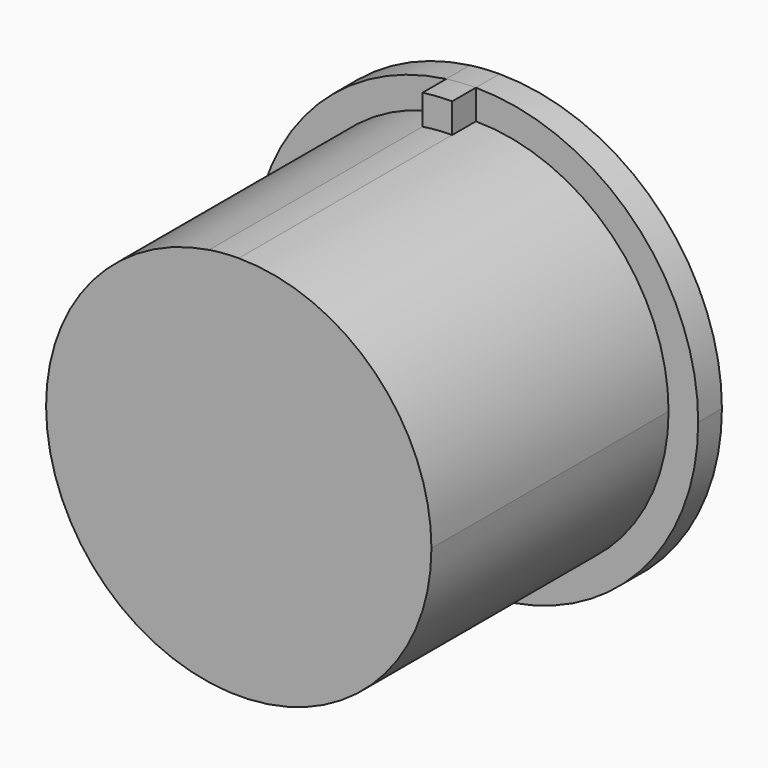
from build123d import *
from build123d import SkipClean  # not in build123d's __all__

# Parameters (mm, degrees)
F3_DEPTH = 3.175
F4_DEPTH = 31.75
F5_DEPTH = 3.175
F6_DEPTH = 3.175


# Not quite as in the source:
# - a length typed as a fraction of an inch, garbled in the dataset ("3 / 203.2 mm" for 3/8 in), is restored


with BuildPart() as f3:
    # F2 (on Front) → F3 (new body)
    with BuildSketch(Plane.XZ):
        with BuildLine():
            Line((-3.175, 23.5998841364), (-3.175, 20.3918067186))
            ThreePointArc((-3.175, 20.3918067186), (-1.5922460699, 20.5759849996), (0, 20.6375))
            Line((0, 20.6375), (0, 23.8125))
            ThreePointArc((0, 23.8125), (-1.591055507, 23.7592865765), (-3.175, 23.5998841364))
        make_face()
        with BuildLine():
            ThreePointArc((20.6375, 0), (-13.4235305294, -15.6753065161), (-3.175, 20.3918067186))
            Line((-3.175, 20.3918067186), (-3.175, 23.5998841364))
            ThreePointArc((-3.175, 23.5998841364), (-15.6753065161, -17.9253987926), (23.8125, 0))
            ThreePointArc((23.8125, 0), (16.837980227, 16.837980227), (0, 23.8125))
            Line((0, 23.8125), (0, 20.6375))
            ThreePointArc((0, 20.6375), (14.5929161967, 14.5929161967), (20.6375, 0))
        make_face()
    extrude(amount=-F3_DEPTH)

    # F2 (on Front) → F4 (join)
    with BuildSketch(Plane.XZ):
        with BuildLine():
            ThreePointArc((0, 20.6375), (-1.5922460699, 20.5759849996), (-3.175, 20.3918067186))
            ThreePointArc((-3.175, 20.3918067186), (-13.4235305294, -15.6753065161), (20.6375, 0))
            ThreePointArc((20.6375, 0), (14.5929161967, 14.5929161967), (0, 20.6375))
        make_face()
    extrude(amount=F4_DEPTH)

    # F2 (on Front) → F5 (join)
    with BuildSketch(Plane.XZ):
        with BuildLine():
            Line((-3.175, 23.5998841364), (-3.175, 20.3918067186))
            ThreePointArc((-3.175, 20.3918067186), (-1.5922460699, 20.5759849996), (0, 20.6375))
            Line((0, 20.6375), (0, 23.8125))
            ThreePointArc((0, 23.8125), (-1.591055507, 23.7592865765), (-3.175, 23.5998841364))
        make_face()
    with SkipClean():  # cleaning this boolean's faces spoils the solid; the shape is the same uncleaned
        extrude(amount=F5_DEPTH)

    # F2 (on Front) → F6 (join)
    with BuildSketch(Plane.XZ):
        with BuildLine():
            ThreePointArc((0, 20.6375), (-1.5922460699, 20.5759849996), (-3.175, 20.3918067186))
            ThreePointArc((-3.175, 20.3918067186), (-13.4235305294, -15.6753065161), (20.6375, 0))
            ThreePointArc((20.6375, 0), (14.5929161967, 14.5929161967), (0, 20.6375))
        make_face()
        with BuildLine():
            Line((-3.175, 23.5998841364), (-3.175, 20.3918067186))
            ThreePointArc((-3.175, 20.3918067186), (-1.5922460699, 20.5759849996), (0, 20.6375))
            Line((0, 20.6375), (0, 23.8125))
            ThreePointArc((0, 23.8125), (-1.591055507, 23.7592865765), (-3.175, 23.5998841364))
        make_face()
    with SkipClean():  # cleaning this boolean's faces spoils the solid; the shape is the same uncleaned
        extrude(amount=-F6_DEPTH)


solid = f3.part
